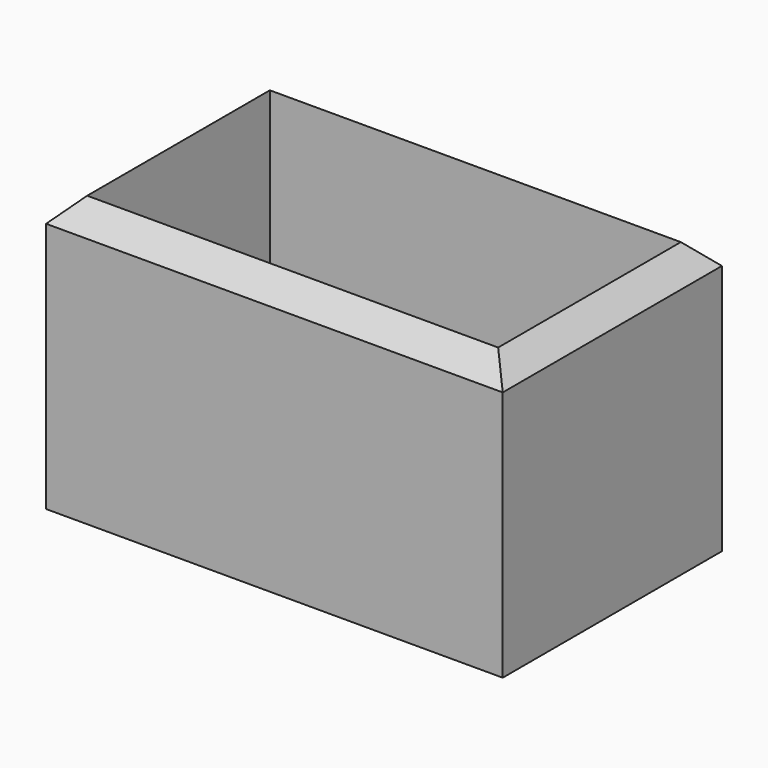
from build123d import *

# Parameters (mm, degrees)
F0_W     = 127
F0_H     = 76.2
F1_DEPTH = 76.2
F2_T     = -6.35
F3_SIZE  = 6.34999


# Not quite as in the source:
# - a fillet or chamfer is up to 0.001 mm smaller than in the source, because OpenCascade refuses the exact size


with BuildPart() as f1:
    # F0 (on Top) → F1 (new body)
    with BuildSketch(Plane.XY):
        with Locations((1.4040806768, -11.3298352808)):
            Rectangle(F0_W, F0_H)
    extrude(amount=F1_DEPTH)

    # F2
    f2_openings = [f1.faces().sort_by_distance(p)[0] for p in [
        (1.404081, -11.329835, 76.2),
    ]]
    offset(amount=F2_T, openings=f2_openings)

    # F3 (size 6.35 in the source; OpenCascade refuses exactly that, so slightly less here)
    f3_edges = [f1.edges().sort_by_distance(p)[0] for p in [
        (1.404081, -49.429835, 76.2),
        (1.404081, 26.770165, 76.2),
        (64.904081, -11.329835, 76.2),
        (-62.095919, -11.329835, 76.2),
    ]]
    chamfer(f3_edges, length=F3_SIZE)


solid = f1.part
